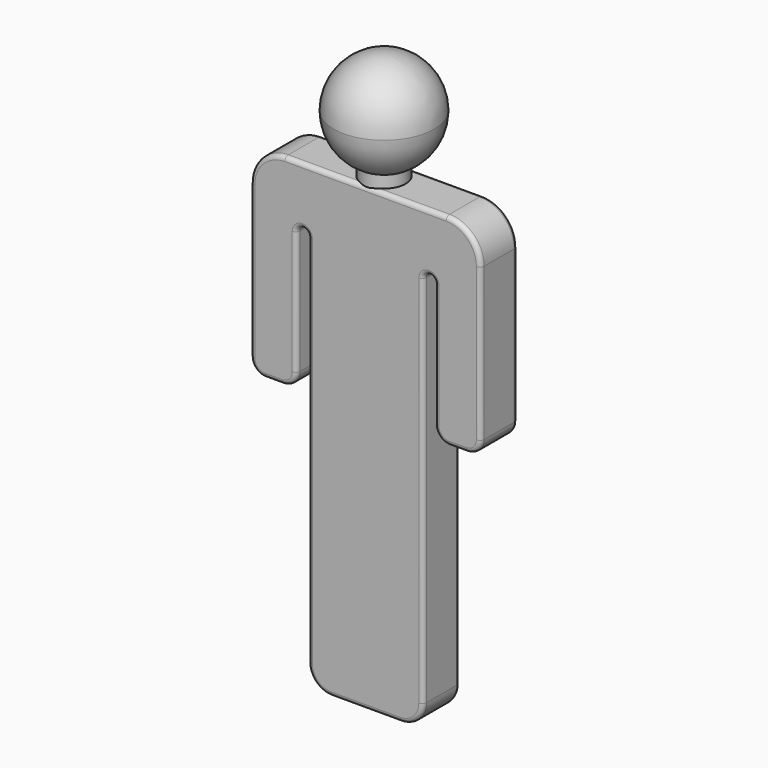
from build123d import *

# Parameters (mm, degrees)
F0_W      = 400
F0_H      = 200
F0_H_2    = 1400
F0_W_2    = 160
F0_H_3    = 500
F1_DEPTH  = 80
F2_R      = 120
F3_R      = 50
F4_R      = 19.99999
F5_R      = 80
F6_R      = 15
F9_R      = 75
F10_DEPTH = 50


# Not quite as in the source:
# - a fillet or chamfer is up to 0.001 mm smaller than in the source, because OpenCascade refuses the exact size


with BuildPart() as f1:
    # F0 (on Front) → F1 (new body, symmetric)
    with BuildSketch(Plane.XZ):
        with Locations((-106.6726207733, 600)):
            Rectangle(F0_W, F0_H)
        Polygon((-306.6726207733, 500), (-306.6726207733, 700), (-506.6726207733, 700), (-506.6726207733, 500), (-346.6726207733, 500), align=None)
        Polygon((293.3273792267, 700), (93.3273792267, 700), (93.3273792267, 500), (133.3273792267, 500), (293.3273792267, 500), align=None)
        with Locations((-106.6726207733, -200)):
            Rectangle(F0_W, F0_H_2)
        with Locations((-426.6726207733, 250)):
            Rectangle(F0_W_2, F0_H_3)
        with Locations((213.3273792267, 250)):
            Rectangle(F0_W_2, F0_H_3)
    extrude(amount=F1_DEPTH, both=True)

    # F2
    f2_edges = [f1.edges().sort_by_distance(p)[0] for p in [
        (293.327379, 0, 700),
        (-506.672621, 0, 700),
    ]]
    fillet(f2_edges, radius=F2_R)

    # F3
    f3_edges = [f1.edges().sort_by_distance(p)[0] for p in [
        (293.327379, 0, 0),
        (-346.672621, 0, 0),
        (133.327379, 0, 0),
        (-506.672621, 0, 0),
    ]]
    fillet(f3_edges, radius=F3_R)

    # F4 (radius 20 in the source; OpenCascade refuses exactly that, so slightly less here)
    f4_edges = [f1.edges().sort_by_distance(p)[0] for p in [
        (-346.672621, 0, 500),
        (93.327379, 0, 500),
        (-306.672621, 0, 500),
        (133.327379, 0, 500),
    ]]
    fillet(f4_edges, radius=F4_R)

    # F5
    f5_edges = [f1.edges().sort_by_distance(p)[0] for p in [
        (-306.672621, 0, -900),
        (93.327379, 0, -900),
    ]]
    fillet(f5_edges, radius=F5_R)

    # F6
    f6_edges = [f1.edges().sort_by_distance(p)[0] for p in [
        (-106.672621, -80, 700),
        (93.327379, 80, -169.999995),
    ]]
    fillet(f6_edges, radius=F6_R)


with BuildPart() as f8:
    # F7 (on Front) → F8 (revolve)
    with BuildSketch(Plane.XZ):
        with BuildLine():
            ThreePointArc((-106.6726207733, 725), (17.0710659343, 776.2563132924), (68.3273792267, 900))
            ThreePointArc((68.3273792267, 900), (17.0710659343, 1023.7436867076), (-106.6726207733, 1075))
            Line((-106.6726207733, 1075), (-106.6726207733, 725))
        make_face()
    revolve(axis=Axis((-106.6726207733, 0, 900), (0, 0, 1)))


with BuildPart() as f10:
    # F9 (on face) → F10 (new body, symmetric)
    with BuildSketch(Plane.XY.offset(700)):
        with Locations((-106.6726207733, 0)):
            Circle(F9_R)
    extrude(amount=F10_DEPTH, both=True)


solid = Compound([f1.part, f8.part, f10.part])
